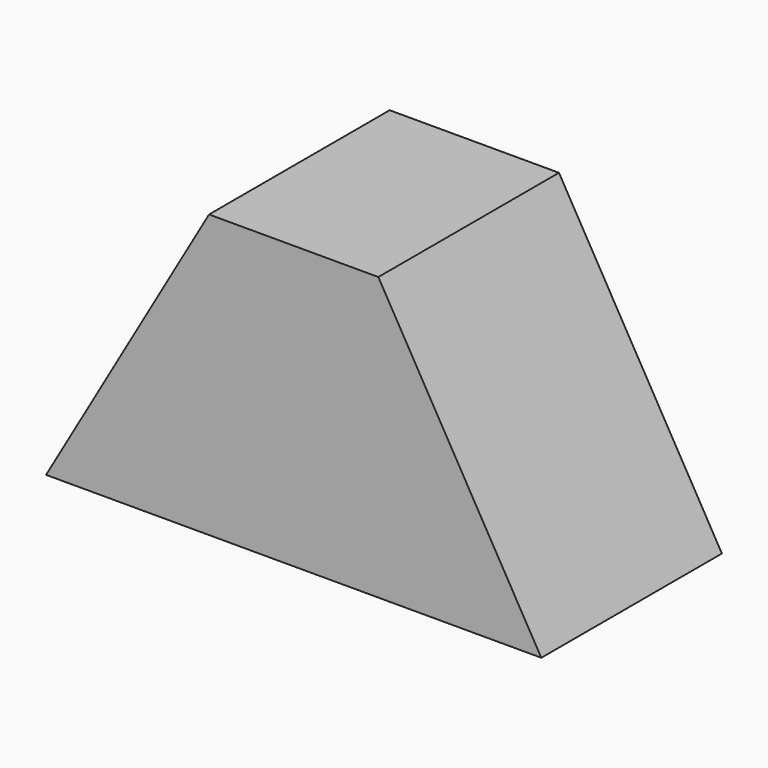
from build123d import *

# Parameters (mm, degrees)
F0_W     = 38.1
F0_H     = 63.5
F1_DEPTH = 25.4
F3_DEPTH = 50.8


# Not quite as in the source:
# - a pattern or mirror of a feature is missing from the dataset's text; its kind, count and spacing are read off the source's solid


with BuildPart() as f1:
    # F0 (on Front) → F1 (new body, symmetric)
    with BuildSketch(Plane.XZ):
        with Locations((0, 31.75)):
            Rectangle(F0_W, F0_H)
    extrude(amount=F1_DEPTH, both=True)

    # F2 (on face) → F3 (join, through all)
    with BuildSketch(Plane.XZ.offset(25.4)):
        Polygon((-19.05, 0), (-19.05, 63.5), (-55.7117420935, 0), align=None)
    f3 = extrude(amount=-F3_DEPTH)

    # F3_copies: F3 across plane
    add(f3.mirror(Plane(origin=(0, 0, 0), x_dir=(0, 0, 1), z_dir=(1, 0, 0))))


solid = f1.part
